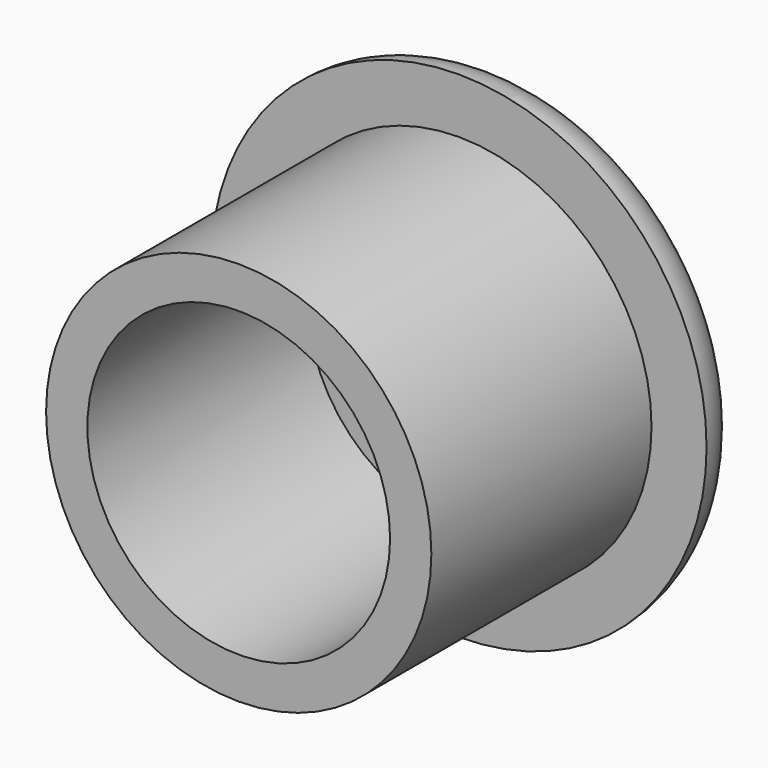
from build123d import *

# Parameters (mm, degrees)
F0_R     = 9
F1_DEPTH = 12
F2_R     = 9
F2_R_2   = 7
F3_DEPTH = 10
F4_R     = 5.5
F5_DEPTH = 10
F6_R     = 1.99999


# Not quite as in the source:
# - a fillet or chamfer is up to 0.001 mm smaller than in the source, because OpenCascade refuses the exact size


with BuildPart() as f1:
    # F0 (on Front) → F1 (new body)
    with BuildSketch(Plane.XZ):
        Circle(F0_R)
    extrude(amount=F1_DEPTH)

    # F2 (on face) → F3 (cut)
    with BuildSketch(Plane.XZ.offset(12)):
        Circle(F2_R)
        Circle(F2_R_2, mode=Mode.SUBTRACT)
    extrude(amount=-F3_DEPTH, mode=Mode.SUBTRACT)

    # F4 (on face) → F5 (cut)
    with BuildSketch(Plane.XZ.offset(12)):
        Circle(F4_R)
    extrude(amount=-F5_DEPTH, mode=Mode.SUBTRACT)

    # F6 (radius 2 in the source; OpenCascade refuses exactly that, so slightly less here)
    f6_edges = [f1.edges().sort_by_distance(p)[0] for p in [
        (-9, 0, 0),
    ]]
    fillet(f6_edges, radius=F6_R)


solid = f1.part
